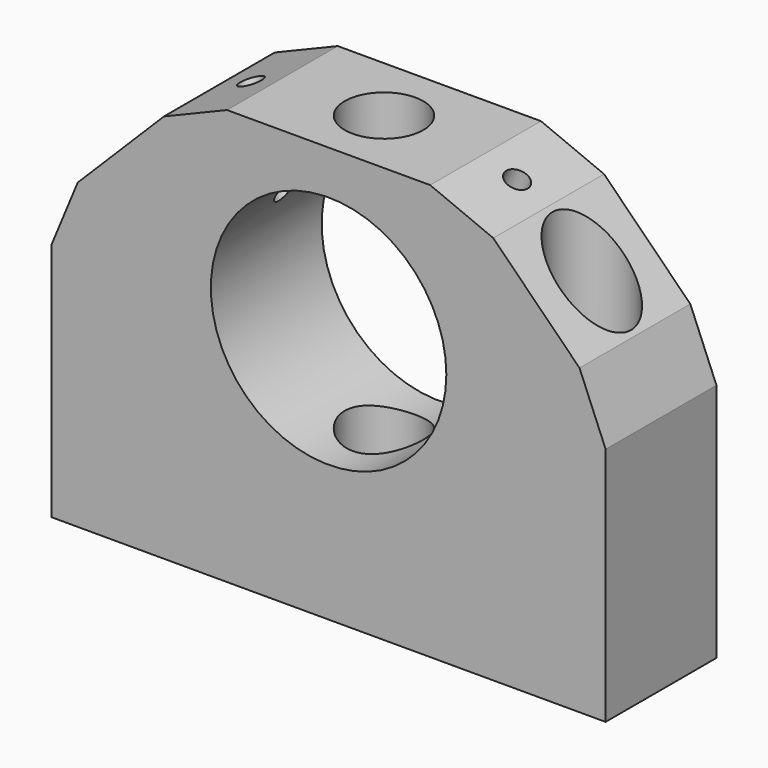
from build123d import *

# Parameters (mm, degrees)
F0_W            = 120
F0_H            = 30
F0_R            = 3.5
F1_DEPTH        = 10
F2_W            = 120
F2_H            = 30
F2_R            = 8.5
F3_DEPTH        = 80
F4_R            = 25.5
F5_DEPTH        = 30
F6_T1_DEPTH     = 184.300979278
F7_SIZE         = 8
F10_D           = 5
F10_DEPTH       = 25
F10_TIP         = 1.5021515476
F10_ON_F9_D     = 5
F10_ON_F9_DEPTH = 25
F10_ON_F9_TIP   = 1.5021515476


# Not quite as in the source:
# - a fillet or chamfer that OpenCascade refuses, or shapes differently, is made with other operations: its cross-section is extruded or revolved along the edge and cut away or added


with BuildPart() as f1:
    # F0 (on Top) → F1 (new body)
    with BuildSketch(Plane.XY):
        with Locations((-5.4327639937, 0)):
            Rectangle(F0_W, F0_H)
        with Locations((-50.4327639937, 0)):
            Circle(F0_R, mode=Mode.SUBTRACT)
        with Locations((-5.4327639937, 0)):
            Circle(F0_R, mode=Mode.SUBTRACT)
        with Locations((39.5672360063, 0)):
            Circle(F0_R, mode=Mode.SUBTRACT)
    extrude(amount=F1_DEPTH)

    # F2 (on face) → F3 (join)
    with BuildSketch(Plane.XY.offset(10)):
        with Locations((-5.4327639937, 0)):
            Rectangle(F2_W, F2_H)
        with Locations((-50.4327639937, 0)):
            Circle(F2_R, mode=Mode.SUBTRACT)
        with Locations((-5.4327639937, 0)):
            Circle(F2_R, mode=Mode.SUBTRACT)
        with Locations((39.5672360063, 0)):
            Circle(F2_R, mode=Mode.SUBTRACT)
    extrude(amount=F3_DEPTH)

    # F4 (on face) → F5 (cut)
    with BuildSketch(Plane.XZ.offset(15)):
        with Locations((-5.4327639937, 55)):
            Circle(F4_R)
    extrude(amount=-F5_DEPTH, mode=Mode.SUBTRACT)

    # F6: chamfer of 30 on 2 edges, made by hand

    # F6_s2 → F6_t1 (cut)
    with BuildSketch(Plane.XZ.offset(-92.150489639)):
        Polygon((-35.4327639937, 90), (-65.4327639937, 60), (-65.4327639937, 90), align=None)
        Polygon((54.5672360063, 60), (24.5672360063, 90), (54.5672360063, 90), align=None)
    extrude(amount=F6_T1_DEPTH, mode=Mode.SUBTRACT)

    # F7
    f7_edges = [f1.edges().sort_by_distance(p)[0] for p in [
        (-65.432764, 0, 60),
        (-35.432764, 0, 90),
        (24.567236, 0, 90),
        (54.567236, 0, 60),
    ]]
    chamfer(f7_edges, length=F7_SIZE)

    # F10
    with Locations(Plane(origin=(-35.8372404269, 0, 86.5187518767), x_dir=(0.9238795325, 0, 0.3826834324), z_dir=(-0.3826834324, 0, 0.9238795325))):
        with Locations((1.7059034787, 0)):
            Hole(F10_D / 2, depth=F10_DEPTH)
            with Locations((0, 0, -(F10_DEPTH + F10_TIP / 2))):  # 118° drill point
                Cone(0, F10_D / 2, F10_TIP, mode=Mode.SUBTRACT)

    # F10 on F9
    with Locations(Plane(origin=(34.2460206938, 0, 82.6772076162), x_dir=(0.9238795325, 0, -0.3826834324), z_dir=(0.3826834324, 0, 0.9238795325))):
        with Locations((-11.7443423963, 0)):
            Hole(F10_ON_F9_D / 2, depth=F10_ON_F9_DEPTH)
            with Locations((0, 0, -(F10_ON_F9_DEPTH + F10_ON_F9_TIP / 2))):  # 118° drill point
                Cone(0, F10_ON_F9_D / 2, F10_ON_F9_TIP, mode=Mode.SUBTRACT)


solid = f1.part
